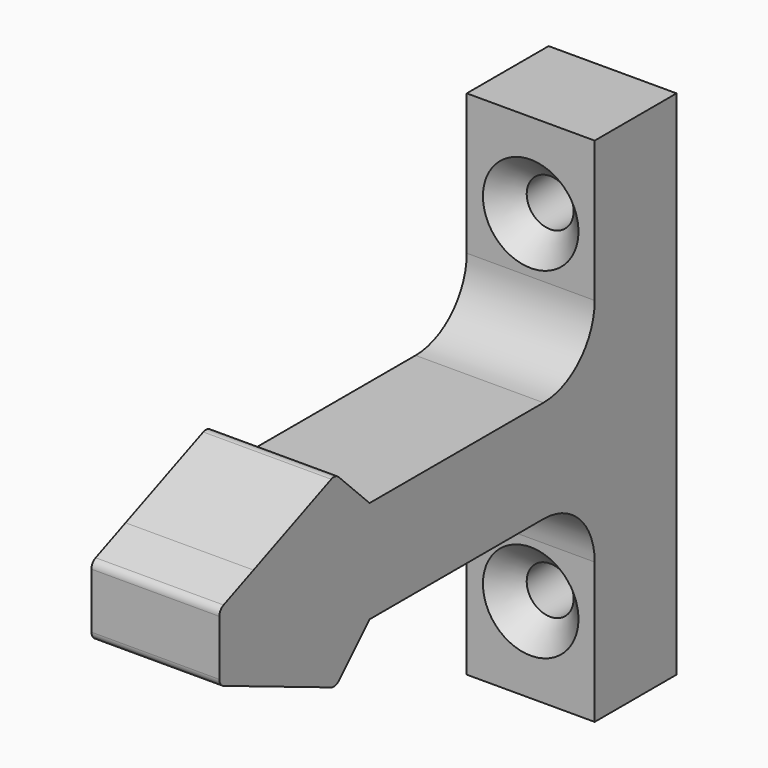
from build123d import *

# Parameters (mm, degrees)
F1_DEPTH       = 7.5
F2_R           = 1
F4_D           = 5.5
F4_CSINK_D     = 11.2
F4_CSINK_ANGLE = 90
F5_R           = 7.5


with BuildPart() as f1:
    # F0 (on Right) → F1 (new body, symmetric)
    with BuildSketch(Plane.YZ):
        Polygon((-67, 0), (-62, 0), (-62, 6), (-67, 3.917779892), align=None)
        Polygon((-62, 6), (-44.9935843937, 6), (-49.9935843937, 11), align=None)
        Polygon((-12, 0), (-12, 6), (-44.9935843937, 6), (-62, 6), (-62, 0), align=None)
        Polygon((-62, -6), (-62, 0), (-67, 0), (-67, -3.917779892), align=None)
        Polygon((-49.9935843937, -11), (-44.9935843937, -6), (-62, -6), align=None)
        Polygon((-12, -6), (-12, 0), (-62, 0), (-62, -6), (-44.9935843937, -6), align=None)
        Polygon((0, 0), (0, 30), (-12, 30), (-12, 6), (-12, 0), align=None)
        Polygon((0, -30), (0, 0), (-12, 0), (-12, -6), (-12, -30), align=None)
    extrude(amount=F1_DEPTH, both=True)

    # F2
    f2_edges = [f1.edges().sort_by_distance(p)[0] for p in [
        (0, -49.993584, 11),
        (0, -67, 3.91778),
        (0, -67, -3.91778),
        (0, -49.993584, -11),
    ]]
    fillet(f2_edges, radius=F2_R)

    # F4 (through all)
    with Locations(Plane.XZ.offset(12)):
        with Locations((0, 20), (0, -20)):
            CounterSinkHole(F4_D / 2, F4_CSINK_D / 2, counter_sink_angle=F4_CSINK_ANGLE)

    # F5
    f5_edges = [f1.edges().sort_by_distance(p)[0] for p in [
        (0, -12, 6),
        (0, -12, -6),
    ]]
    fillet(f5_edges, radius=F5_R)


solid = f1.part
